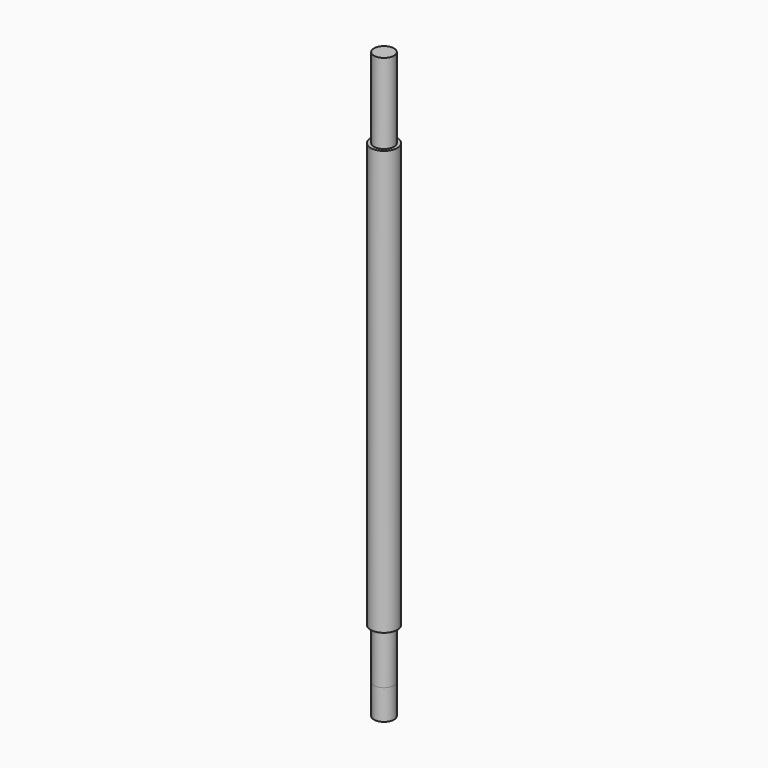
from build123d import *

# Parameters (mm, degrees)
F2_DEPTH = 9
F3_DEPTH = 9


with BuildPart() as f1:
    # F0 (on Front) → F1 (revolve)
    with BuildSketch(Plane.XZ):
        Polygon((0, -50), (0, 107), (-3, 107), (-3, 92), (-4, 92), (-4, -35), (-3, -35), (-3, -50), align=None)
    revolve(axis=Axis((0, 0, 0), (0, 0, -1)))

    # F2 (add): a face of the model
    f2_faces = [f1.faces().sort_by_distance(p)[0] for p in [
        (0, 0, 107),
    ]]
    extrude(f2_faces, amount=F2_DEPTH)

    # F3 (add): a face of the model
    f3_faces = [f1.faces().sort_by_distance(p)[0] for p in [
        (0, 0, -50),
    ]]
    extrude(f3_faces, amount=F3_DEPTH)


solid = f1.part
